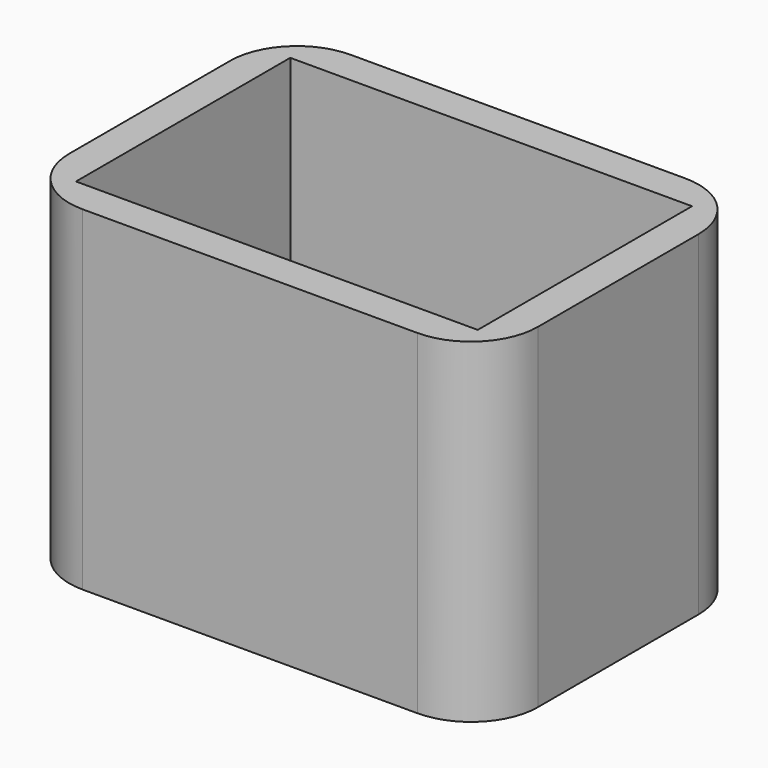
from build123d import *

# Parameters (mm, degrees)
F0_W     = 177.8
F0_H     = 127
F1_DEPTH = 127
F2_T     = -12.7
F3_DEPTH = 25.4
F4_R     = 25.4


with BuildPart() as f1:
    # F0 (on Top) → F1 (new body)
    with BuildSketch(Plane.XY):
        with Locations((88.9, -63.5)):
            Rectangle(F0_W, F0_H)
    extrude(amount=F1_DEPTH)

    # F2
    f2_openings = [f1.faces().sort_by_distance(p)[0] for p in [
        (88.9, -63.5, 127),
    ]]
    offset(amount=F2_T, openings=f2_openings)

    # F3 (add): a face of the model
    f3_faces = [f1.faces().sort_by_distance(p)[0] for p in [
        (88.9, -63.5, 12.7),
    ]]
    extrude(f3_faces, amount=F3_DEPTH)

    # F4
    f4_edges = [f1.edges().sort_by_distance(p)[0] for p in [
        (177.8, 0, 63.5),
        (177.8, -127, 63.5),
        (0, 0, 63.5),
        (0, -127, 63.5),
    ]]
    fillet(f4_edges, radius=F4_R)


solid = f1.part
